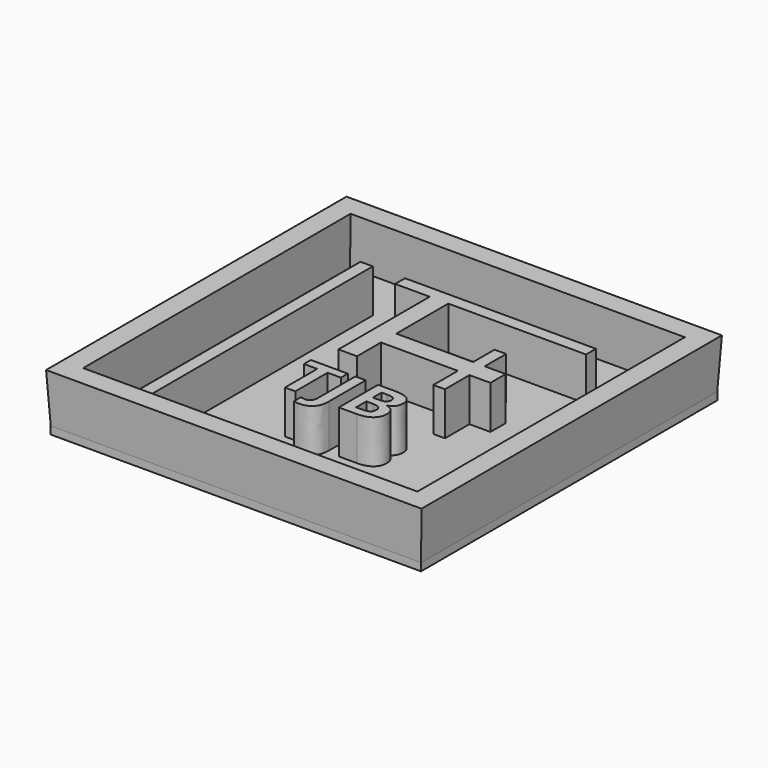
from build123d import *

# Parameters (mm, degrees)
F0_W         = 38.1
F0_H         = 38.1
F1_DEPTH     = 0.79375
F2_W         = 38.1
F2_H         = 38.1
F2_W_2       = 34.925
F2_H_2       = 34.925
F3_DEPTH     = 5.08
F3_TAPER     = -3
F4_R         = 1.27
F5_DEPTH     = 0.396875
F4_W         = 1.27
F4_H         = 29.5787684812
F6_DEPTH     = 4.445
F4_TEXT_SIZE = 7.0555555556
F7_DEPTH     = 4.445


# Not quite as in the source:
# - Text() gives the source's letters only with a copy of the font that has no kerning and outlines rounded to 1/6400 em; it was checked with that copy


with BuildPart() as f1:
    # F0 (on Top) → F1 (new body)
    with BuildSketch(Plane.XY):
        with Locations((-3.8427002728, -0.7210307556)):
            Rectangle(F0_W, F0_H)
    extrude(amount=F1_DEPTH)

    # F2 (on face) → F3 (join)
    with BuildSketch(Plane.XY.offset(0.79375)):
        with Locations((-3.8427002728, -0.7210307556)):
            Rectangle(F2_W, F2_H)
        with Locations((-3.8427002728, -0.7210307556)):
            Rectangle(F2_W_2, F2_H_2, mode=Mode.SUBTRACT)
    extrude(amount=F3_DEPTH, taper=F3_TAPER)

    # F4 (on face) → F5 (cut)
    with BuildSketch(Plane.XY.offset(0.79375)):
        with Locations((-18.6320845134, -13.9806950465)):
            Circle(F4_R)
        with Locations((-12.1261980385, -14.7828003392)):
            Circle(F4_R)
    extrude(amount=-F5_DEPTH, mode=Mode.SUBTRACT)

    # F4 (on face) → F6 (join)
    with BuildSketch(Plane.XY.offset(0.79375)):
        with Locations((-15.323968754, -3.394146515)):
            Rectangle(F4_W, F4_H)
        Polygon((8.2735682084, 11.3952377256), (-11.3735990599, 11.3952377256), (-11.3735990599, 10.1252377256), (-7.8150574118, 10.1252377256), (-7.8150574118, -1.6126377983), (-5.9030051343, -1.6126377983), (-5.9030051343, 1.4678905475), (2.0054364577, 1.4678905475), (2.0054364577, -1.6814563423), (3.1977731269, -1.6814563423), (3.1977731269, 1.4678905475), (5.3568566218, 1.4678905475), (5.3568566218, 3.4330552201), (3.1977731269, 3.4330552201), (3.1977731269, 6.1879656278), (2.0054364577, 6.1879656278), (2.0054364577, 3.4330552201), (-5.9030051343, 3.4330552201), (-5.9030051343, 10.1252377256), (8.2735682084, 10.1252377256), align=None)
    extrude(amount=F6_DEPTH)

    # F4 (on face) → F7 (join)
    with BuildSketch(Plane.XY.offset(0.79375)):
        with Locations((-8.5394951748, -9.4727775278)):
            Text('TJB', F4_TEXT_SIZE, font='Open Sans', font_style=FontStyle.BOLD, text_align=(TextAlign.LEFT, TextAlign.BOTTOM))
    extrude(amount=F7_DEPTH)


solid = f1.part
